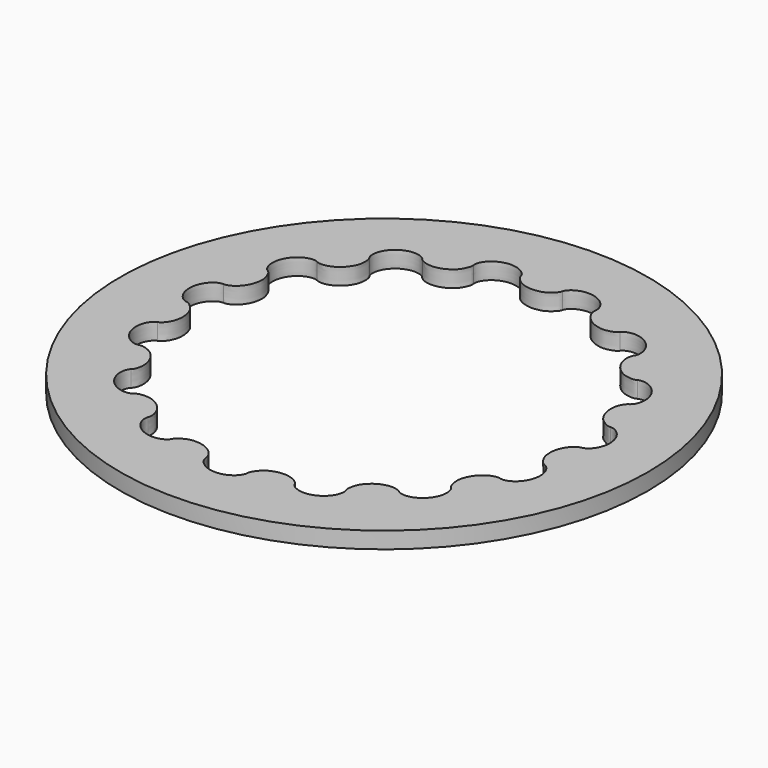
from build123d import *

# Parameters (mm, degrees)
F1_R            = 40
F1_R_2          = 30
F2_DEPTH        = 2.5
F4_DEPTH        = 2.5
F4_COPIES_COUNT = 15
F6_DEPTH        = 2.5
F6_COPIES_COUNT = 15


# Not quite as in the source:
# - a pattern or mirror of a feature is missing from the dataset's text; its kind, count and spacing are read off the source's solid


with BuildPart() as f2:
    # F1 (on Top) → F2 (new body)
    with BuildSketch(Plane.XY):
        Circle(F1_R)
        Circle(F1_R_2, mode=Mode.SUBTRACT)
    extrude(amount=F2_DEPTH)

    # F3 (on face) → F4 (cut, through all)
    with BuildSketch(Plane.XY.offset(2.5)):
        with BuildLine():
            add(Edge.make_bspline(
                [(29.344428022, 6.2373507245), (29.3933354021, 6.2477463091), (29.4907818104, 6.2458927428), (29.9260713153, 6.1668744849), (30.4933926149, 5.8549659014), (31.1158428866, 5.2590115229), (31.614702741, 4.3921350903), (31.874991761, 3.3501963002), (31.8370218419, 2.2769099498), (31.5292969648, 1.3252579493), (31.0443549487, 0.6129120372), (30.5542793765, 0.189866424), (30.1449362259, 0.0220748714), (30.049999975, 0), (30, 4.9956e-05)],
                knots=[0, 0, 0, 0, 0.0392231241, 0.1063510743, 0.1910134394, 0.2876620616, 0.3919582226, 0.5000006598, 0.6080430653, 0.7123392263, 0.8089878485, 0.8936502136, 0.9607781638, 1, 1, 1, 1], degree=3))
            ThreePointArc((29.344428022, 6.2373507245), (29.3977411386, 5.9810380325), (29.4488155034, 5.7242698613))
            ThreePointArc((29.4488155034, 5.7242698613), (29.4976472269, 5.4670657648), (29.5442325904, 5.20944533))
            ThreePointArc((29.5442325904, 5.20944533), (29.8858387658, 2.6146971654), (30, 4.9956e-05))
        make_face()
    f4 = extrude(amount=-F4_DEPTH, mode=Mode.SUBTRACT)

    # F4_copies: F4 ×15 about axis
    f4_copies_axis = Axis((0, 0, 0), (0, 0, 1))
    for i in range(1, F4_COPIES_COUNT):
        add(f4.rotate(f4_copies_axis, i * 360 / F4_COPIES_COUNT), mode=Mode.SUBTRACT)

    # F5 (on face) → F6 (join, through all)
    with BuildSketch(Plane.XY.offset(2.5)):
        with BuildLine():
            ThreePointArc((27.6151456036, 11.7219338547), (27.5118022316, 11.9624720678), (27.4063637293, 12.2020992923))
            add(Edge.make_bspline(
                [(29.344428022, 6.2373507245), (29.295520642, 6.22695514), (29.2022743002, 6.233123582), (28.7746198394, 6.2419232171), (27.5472761579, 6.9892563869), (27.043052587, 7.71669433), (26.5824231035, 8.6436931859), (26.4014788587, 9.6227803042), (26.4464444164, 10.5561239597), (26.685775911, 11.3246501923), (26.9886897968, 11.8453432179), (27.2921046088, 12.1314608661), (27.3606864564, 12.1817624601), (27.4063637293, 12.2020992923)],
                knots=[0, 0, 0, 0, 0.0414260396, 0.1123321793, 0.2475649801, 0.3577326485, 0.4718575381, 0.5859823857, 0.6961500541, 0.7982395608, 0.8876678207, 0.9585739604, 1, 1, 1, 1], degree=3))
            ThreePointArc((29.344428022, 6.2373507245), (28.6115085224, 9.0211739851), (27.6151456036, 11.7219338547))
        make_face()
    f6 = extrude(amount=-F6_DEPTH)

    # F6_copies: F6 ×15 about axis
    f6_copies_axis = Axis((0, 0, 0), (0, 0, 1))
    for i in range(1, F6_COPIES_COUNT):
        add(f6.rotate(f6_copies_axis, i * 360 / F6_COPIES_COUNT))


solid = f2.part
